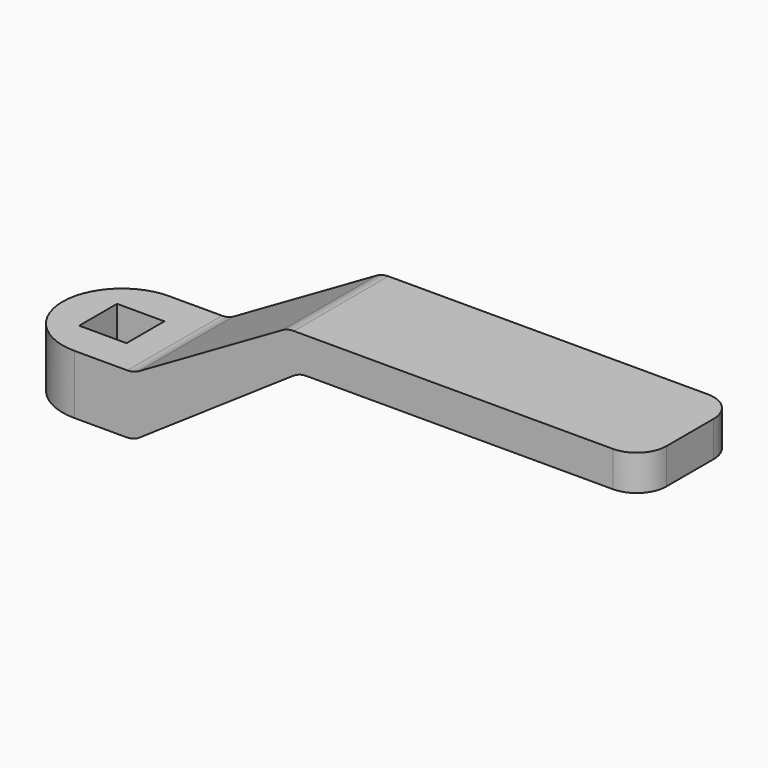
from build123d import *

# Parameters (mm, degrees)
F1_DEPTH = 10
F2_W     = 8
F2_H     = 8
F3_DEPTH = 10
F4_R     = 9.99999
F5_R     = 4
F6_R     = 5


# Not quite as in the source:
# - a fillet or chamfer is up to 0.001 mm smaller than in the source, because OpenCascade refuses the exact size


with BuildPart() as f1:
    # F0 (on Front) → F1 (new body, symmetric)
    with BuildSketch(Plane.XZ):
        Polygon((35.9807621135, 20), (10, 5), (-10, 5), (-10, -5), (10, -5), (37.9807621135, 14), (95.9807621135, 14), (95.9807621135, 20), align=None)
    extrude(amount=F1_DEPTH, both=True)

    # F2 (on face) → F3 (cut, through all)
    with BuildSketch(Plane.XY.offset(5)):
        Rectangle(F2_W, F2_H)
    extrude(amount=-F3_DEPTH, mode=Mode.SUBTRACT)

    # F4 (radius 10 in the source; OpenCascade refuses exactly that, so slightly less here)
    f4_edges = [f1.edges().sort_by_distance(p)[0] for p in [
        (-10, -10, 0),
        (-10, 10, 0),
    ]]
    fillet(f4_edges, radius=F4_R)

    # F5
    f5_edges = [f1.edges().sort_by_distance(p)[0] for p in [
        (35.980762, 0, 20),
        (10, 0, 5),
        (10, 0, -5),
        (37.980762, 0, 14),
    ]]
    fillet(f5_edges, radius=F5_R)

    # F6
    f6_edges = [f1.edges().sort_by_distance(p)[0] for p in [
        (95.980762, 10, 17),
        (95.980762, -10, 17),
    ]]
    fillet(f6_edges, radius=F6_R)


solid = f1.part
